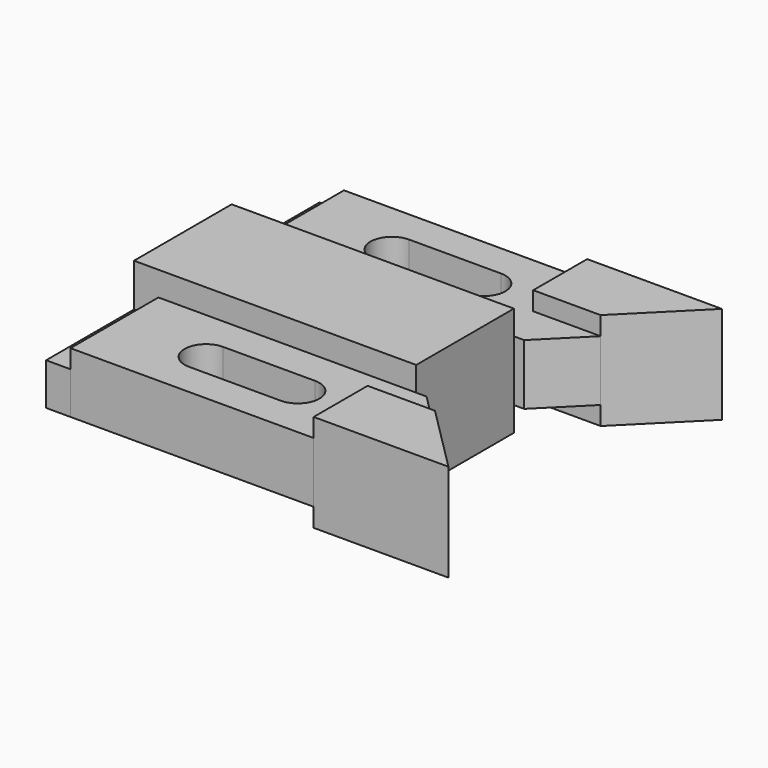
from build123d import *

# Parameters (mm, degrees)
F1_DEPTH = 14.224
F2_DEPTH = 12.7
F3_DEPTH = 7.874
F0_W     = 6.35
F0_H     = 28.575
F4_DEPTH = 7.874
F5_DEPTH = 3.048


with BuildPart() as f1:
    # F0 (on Top) → F1 (new body, symmetric)
    with BuildSketch(Plane.XY):
        Polygon((21.082, 15.875), (-45.974, 15.875), (-52.324, 15.875), (-52.324, -15.875), (-45.974, -15.875), (21.082, -15.875), align=None)
    extrude(amount=F1_DEPTH, both=True)


with BuildPart() as f2:
    # F0 (on Top) → F2 (new body, symmetric)
    with BuildSketch(Plane.XY):
        Polygon((34.798, 26.924), (52.324, 44.45), (17.272, 44.45), (17.272, 26.924), align=None)
    extrude(amount=F2_DEPTH, both=True)


with BuildPart() as f2b:
    # F0 (on Top) → F2, piece 2 (new body, symmetric)
    with BuildSketch(Plane.XY):
        Polygon((52.324, -44.45), (34.798, -26.924), (17.272, -26.924), (17.272, -44.45), align=None)
    extrude(amount=F2_DEPTH, both=True)


with BuildPart() as f3:
    # F0 (on Top) → F3 (new body, symmetric)
    with BuildSketch(Plane.XY):
        Polygon((17.272, 26.924), (17.272, 44.45), (-45.974, 44.45), (-45.974, 15.875), (21.082, 15.875), (23.749, 15.875), (34.798, 26.924), align=None)
        with BuildLine():
            Line((1.778, 24.638), (-22.098, 24.638))
            ThreePointArc((-22.098, 24.638), (-27.686, 30.226), (-22.098, 35.814))
            Line((-22.098, 35.814), (1.778, 35.814))
            ThreePointArc((1.778, 35.814), (7.366, 30.226), (1.778, 24.638))
        make_face(mode=Mode.SUBTRACT)
    extrude(amount=F3_DEPTH, both=True)


with BuildPart() as f3b:
    # F0 (on Top) → F3, piece 2 (new body, symmetric)
    with BuildSketch(Plane.XY):
        Polygon((23.749, -15.875), (21.082, -15.875), (-45.974, -15.875), (-45.974, -44.45), (17.272, -44.45), (17.272, -26.924), (34.798, -26.924), align=None)
        with BuildLine():
            ThreePointArc((-22.098, -35.814), (-27.686, -30.226), (-22.098, -24.638))
            Line((-22.098, -24.638), (1.778, -24.638))
            ThreePointArc((1.778, -24.638), (7.366, -30.226), (1.778, -35.814))
            Line((1.778, -35.814), (-22.098, -35.814))
        make_face(mode=Mode.SUBTRACT)
    extrude(amount=F3_DEPTH, both=True)


with BuildPart() as f4:
    # F0 (on Top) → F4 (new body)
    with BuildSketch(Plane.XY):
        with Locations((-49.149, -30.1625)):
            Rectangle(F0_W, F0_H)
    extrude(amount=-F4_DEPTH)

    # F0 (on Top) → F5, piece 2 (join)
    with BuildSketch(Plane.XY):
        with Locations((-49.149, -30.1625)):
            Rectangle(F0_W, F0_H)
    extrude(amount=F5_DEPTH)


with BuildPart() as f4b:
    # F0 (on Top) → F4, piece 2 (new body)
    with BuildSketch(Plane.XY):
        with Locations((-49.149, 30.1625)):
            Rectangle(F0_W, F0_H)
    extrude(amount=-F4_DEPTH)

    # F0 (on Top) → F5 (join)
    with BuildSketch(Plane.XY):
        with Locations((-49.149, 30.1625)):
            Rectangle(F0_W, F0_H)
    extrude(amount=F5_DEPTH)


solid = Compound([f1.part, f2.part, f2b.part, f3.part, f3b.part, f4.part, f4b.part])
